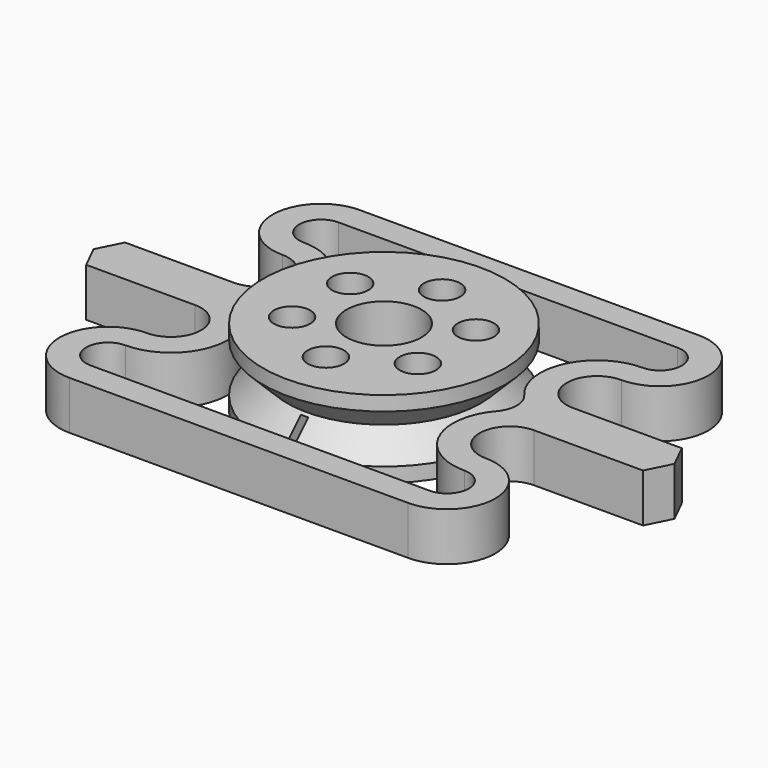
from build123d import *

# Parameters (mm, degrees)
F1_DEPTH = 4
F4_R     = 1.5
F4_R_2   = 1.4
F5_DEPTH = 6.401
F4_R_3   = 3.1
F6_DEPTH = 4
F8_DEPTH = 3


# Not quite as in the source:
# - a feature names something its author has since deleted; it is built from what else it names


with BuildPart() as f1:
    # F0 (on Top) → F1 (new body)
    with BuildSketch(Plane.XY):
        with BuildLine():
            Line((-23, 2), (-24, 0))
            Line((-24, 0), (-23, -2))
            Line((-23, -2), (-14, -2))
            ThreePointArc((-14, -2), (-11.5, -4.5), (-14, -7))
            ThreePointArc((-14, -7), (-18, -11), (-14, -15))
            Line((-14, -15), (0, -15))
            Line((0, -15), (14, -15))
            ThreePointArc((14, -15), (18, -11), (14, -7))
            ThreePointArc((14, -7), (11.5, -4.5), (14, -2))
            Line((14, -2), (23, -2))
            Line((23, -2), (24, 0))
            Line((24, 0), (23, 2))
            Line((23, 2), (14, 2))
            ThreePointArc((14, 2), (11.5, 4.5), (14, 7))
            ThreePointArc((14, 7), (18, 11), (14, 15))
            Line((14, 15), (0, 15))
            Line((0, 15), (-14, 15))
            ThreePointArc((-14, 15), (-18, 11), (-14, 7))
            ThreePointArc((-14, 7), (-11.5, 4.5), (-14, 2))
            Line((-14, 2), (-23, 2))
        make_face()
        with BuildLine():
            ThreePointArc((-14, -9.2000002265), (-9.7282015038, -6.4600356469), (-10.4370736488, -1.4347825616))
            ThreePointArc((-10.4370736488, -1.4347825616), (-10.969320969, 0), (-10.4370736488, 1.4347825616))
            ThreePointArc((-10.4370736488, 1.4347825616), (-9.7282015038, 6.4600356469), (-14, 9.2000002265))
            ThreePointArc((-14, 9.2000002265), (-15.7999997735, 11), (-14, 12.7999997735))
            Line((-14, 12.7999997735), (0.5136036673, 12.7999997735))
            Line((0.5136036673, 12.7999997735), (14, 12.7999997735))
            ThreePointArc((14, 12.7999997735), (15.7999997735, 11), (14, 9.2000002265))
            ThreePointArc((14, 9.2000002265), (9.7282015038, 6.4600356469), (10.4370736488, 1.4347825616))
            ThreePointArc((10.4370736488, 1.4347825616), (10.969320969, 0), (10.4370736488, -1.4347825616))
            ThreePointArc((10.4370736488, -1.4347825616), (9.7282015038, -6.4600356469), (14, -9.2000002265))
            ThreePointArc((14, -9.2000002265), (15.7999997735, -11), (14, -12.7999997735))
            Line((14, -12.7999997735), (0, -12.7999997735))
            Line((0, -12.7999997735), (-14, -12.7999997735))
            ThreePointArc((-14, -12.7999997735), (-15.7999997735, -11), (-14, -9.2000002265))
        make_face(mode=Mode.SUBTRACT)
    extrude(amount=F1_DEPTH)


with BuildPart() as f3:
    # F2 (on Front) → F3 (revolve)
    with BuildSketch(Plane.XZ):
        Polygon((0, 6.4), (0, 0), (10, 0), (10, 1.2), (8, 3.2), (10, 5.2), (10, 6.4), align=None)
    revolve(axis=Axis((0, 0, 3.2), (0, 0, -1)))

    # F4 (on face) → F5 (cut, through all)
    with BuildSketch(Plane.XY.offset(6.4)):
        with Locations((5.1961524227, 3)):
            Circle(F4_R)
        with Locations((5.1961524227, -3)):
            Circle(F4_R)
        with Locations((0, -6)):
            Circle(F4_R)
        with Locations((-5.1961524227, -3)):
            Circle(F4_R)
        with Locations((-5.1961524227, 3)):
            Circle(F4_R)
        Circle(F4_R_2)
        with Locations((0, 6)):
            Circle(F4_R)
    extrude(amount=-F5_DEPTH, mode=Mode.SUBTRACT)

    # F4 (on face) → F6 (cut)
    with BuildSketch(Plane.XY.offset(6.4)):
        Circle(F4_R_3)
        Circle(F4_R_2, mode=Mode.SUBTRACT)
    extrude(amount=-F6_DEPTH, mode=Mode.SUBTRACT)

    # F7 (on face) → F8 (cut)
    with BuildSketch(Plane(origin=(0, 0, 0), x_dir=(1, 0, 0), z_dir=(0, 0, -1))):
        with BuildLine():
            ThreePointArc((-0.3, 7.4696938457), (0, 7.5), (0.3, 7.4696938457))
            Line((0.3, 7.4696938457), (0.3, 9.995498987))
            ThreePointArc((0.3, 9.995498987), (0, 10), (-0.3, 9.995498987))
            Line((-0.3, 9.995498987), (-0.3, 7.4696938457))
        make_face()
    extrude(amount=-F8_DEPTH, mode=Mode.SUBTRACT)


solid = Compound([f1.part, f3.part])
